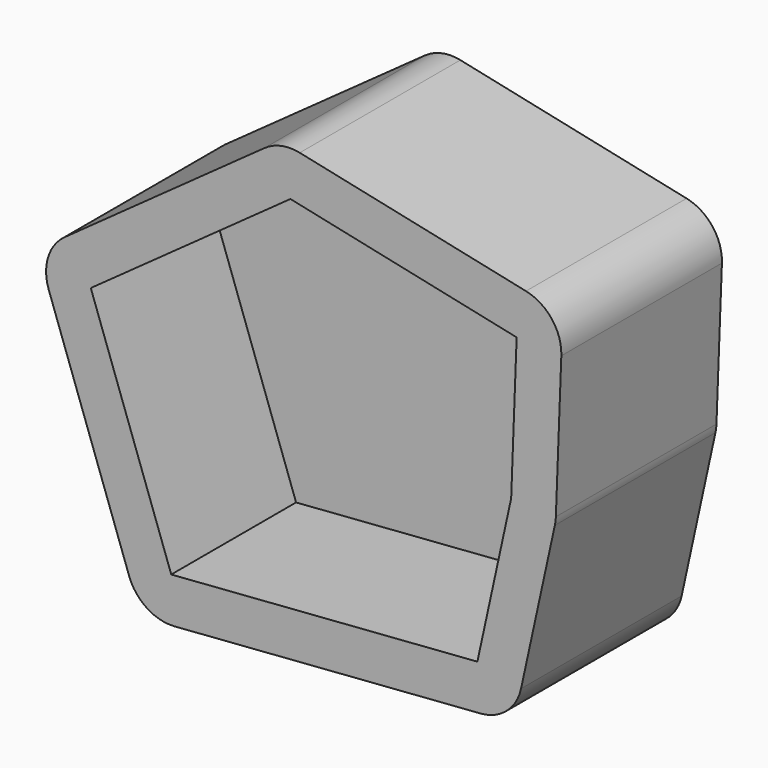
from build123d import *

# Parameters (mm, degrees)
F1_DEPTH = 44.9
F2_T     = 10


# Not quite as in the source:
# - a shell that OpenCascade refuses in one call is made with other operations: the cavity is built on its own and cut out


with BuildPart() as f1:
    # F0 (on Front) → F1 (new body)
    with BuildSketch(Plane.XZ):
        with BuildLine():
            Line((-10.8614214341, 52.2791932931), (-55.5132357346, 20.2294568531))
            ThreePointArc((-55.5132357346, 20.2294568531), (-59.2261437786, 15.0907818347), (-59.1031517936, 8.7522851628))
            Line((-59.1031517936, 8.7522851628), (-41.1086877204, -41.8035860786))
            ThreePointArc((-41.1086877204, -41.8035860786), (-37.1445537144, -46.8302155121), (-30.9441109574, -48.4226575039))
            Line((-30.9441109574, -48.4226575039), (37.5255827113, -43.3174577507))
            ThreePointArc((37.5255827113, -43.3174577507), (43.3388920745, -40.8954764028), (46.5517141249, -35.4789891764))
            Line((46.5517141249, -35.4789891764), (54.1115878941, -0.8666353692))
            ThreePointArc((54.1115878941, -0.8666353692), (54.2619213312, 0.0049565354), (54.334653207, 0.886422737))
            Line((54.334653207, 0.886422737), (55.5578979933, 32.9868546181))
            ThreePointArc((55.5578979933, 32.9868546181), (53.4569722953, 39.5092382704), (47.6504120091, 43.1478142196))
            Line((47.6504120091, 43.1478142196), (-2.9450499877, 53.9354364594))
            ThreePointArc((-2.9450499877, 53.9354364594), (-7.0781470335, 53.9433412691), (-10.8614214341, 52.2791932931))
        make_face()
    extrude(amount=F1_DEPTH)

    # F2: shell of thickness 10, made by hand


with BuildPart() as f2_core1:
    # F2_t2: copy of F1
    add(f1.part)

    # the walls: a layer under each face that stays
    f2_faces = [f2_core1.faces().sort_by_distance(p)[0] for p in [
        (54.9462756001, -22.45, 16.9366386775),
        (22.3526810107, -22.45, 48.5416253395),
        (-33.1873285843, -22.45, 36.2543250731),
        (-50.105919757, -22.45, -16.5256504579),
        (3.2907358769, -22.45, -45.8700576273),
        (50.3316510095, -22.45, -18.1728122728),
        (-2.0584874118, 0, 2.8524646536),
    ]]
    thicken(f2_faces, amount=-F2_T, mode=Mode.SUBTRACT)


with BuildPart() as f1_1:
    add(f1.part)

    # what is left inside the walls is the cavity
    f2_cavity = [f2_core1.part.solids().sort_by_distance(p)[0] for p in [
        (-2.058487, -10.1, -10.915137),
    ]]
    add(f2_cavity, mode=Mode.SUBTRACT)


solid = f1_1.part
